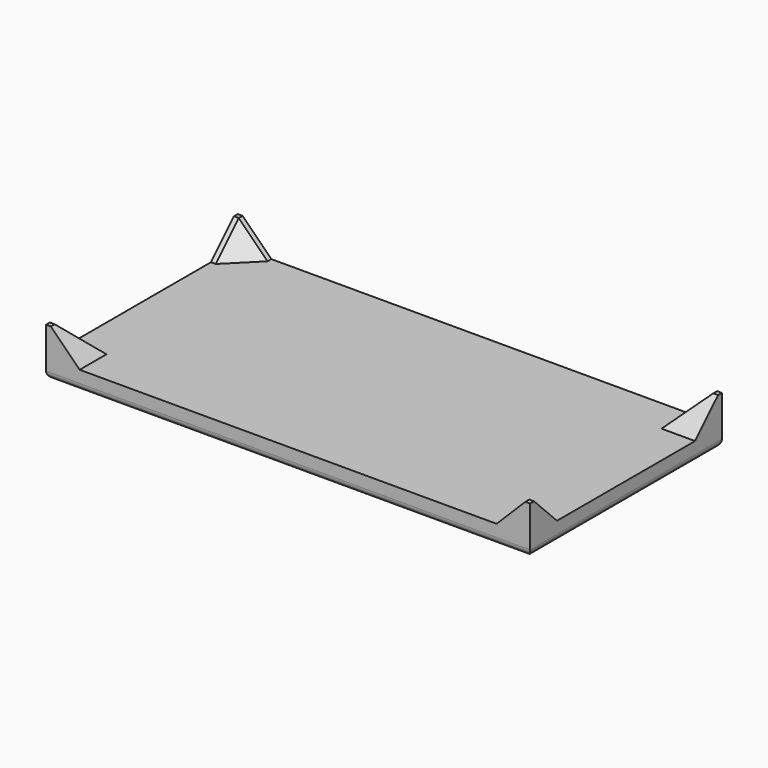
from build123d import *

# Parameters (mm, degrees)
F1_DEPTH = 4
F0_W     = 7
F0_H     = 7
F2_DEPTH = 10
F3_SIZE  = 5.99999
F4_R     = 1.5


# Not quite as in the source:
# - a fillet or chamfer is up to 0.001 mm smaller than in the source, because OpenCascade refuses the exact size


with BuildPart() as f1:
    # F0 (on Top) → F1 (new body)
    with BuildSketch(Plane.XY):
        Polygon((43.5, 25), (-43.5, 25), (-43.5, 18), (-50.5, 18), (-50.5, -18), (-43.5, -18), (-43.5, -25), (43.5, -25), (43.5, -18), (50.5, -18), (50.5, 18), (43.5, 18), align=None)
    extrude(amount=F1_DEPTH)

    # F0 (on Top) → F2 (join)
    with BuildSketch(Plane.XY):
        with Locations((-47, 21.5)):
            Rectangle(F0_W, F0_H)
        with Locations((-47, -21.5)):
            Rectangle(F0_W, F0_H)
        with Locations((47, 21.5)):
            Rectangle(F0_W, F0_H)
        with Locations((47, -21.5)):
            Rectangle(F0_W, F0_H)
    extrude(amount=F2_DEPTH)

    # F3 (size 6 in the source; OpenCascade refuses exactly that, so slightly less here)
    f3_edges = [f1.edges().sort_by_distance(p)[0] for p in [
        (-43.5, 18, 7),
        (-47, 18, 10),
        (-43.5, 21.5, 10),
        (43.5, 21.5, 10),
        (47, 18, 10),
        (47, -18, 10),
        (43.5, -21.5, 10),
        (-43.5, -21.5, 10),
        (-47, -18, 10),
    ]]
    chamfer(f3_edges, length=F3_SIZE)

    # F4
    f4_edges = [f1.edges().sort_by_distance(p)[0] for p in [
        (-50.5, 0, 0),
        (0, -25, 0),
        (50.5, 0, 0),
        (0, 25, 0),
    ]]
    fillet(f4_edges, radius=F4_R)


solid = f1.part
